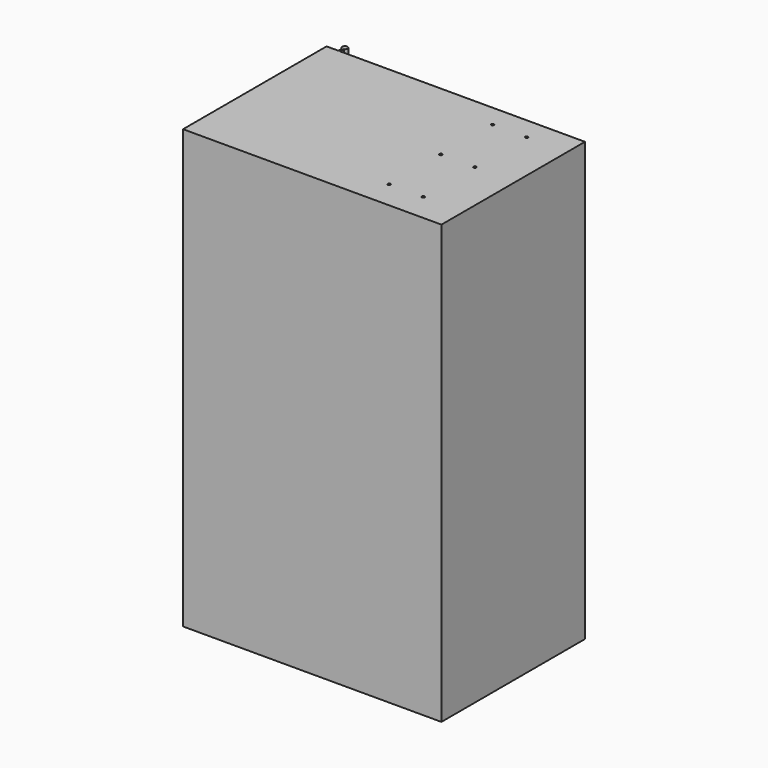
from build123d import *

# Parameters (mm, degrees)
F0_W      = 457.2
F0_H      = 774.7
F1_DEPTH  = 317.5
F2_W      = 381
F2_H      = 698.5
F3_W      = 428.625
F3_H      = 698.5
F4_DEPTH  = 298.45
F5_START  = 19.05
F5_DEPTH  = 279.4
F7_DEPTH  = 774.7
F9_D      = 4.9149
F9_DEPTH  = 38.1
F9_TIP    = 1.4765849282
F10_R     = 2.413
F11_DEPTH = 25.4


# Not quite as in the source:
# - a feature names something its author has since deleted; it is built from what else it names


with BuildPart() as f1:
    # F0 (on Front) → F1 (new body)
    with BuildSketch(Plane.XZ):
        with Locations((0, 387.35)):
            Rectangle(F0_W, F0_H)
    extrude(amount=F1_DEPTH)

    # F2 (on Front) + F3 (on Front) → F4 (cut)
    with BuildSketch(Plane.XZ):
        with Locations((0, 387.35)):
            Rectangle(F2_W, F2_H)
    with BuildSketch(Plane.XZ):
        with Locations((0, 387.35)):
            Rectangle(F3_W, F3_H)
    extrude(amount=F4_DEPTH, mode=Mode.SUBTRACT)

    # F3 (on Front) → F5 (cut)
    with BuildSketch(Plane.XZ.offset(F5_START)):
        with Locations((0, 387.35)):
            Rectangle(F3_W, F3_H)
    extrude(amount=F5_DEPTH, mode=Mode.SUBTRACT)

    # F6 (on Top) → F7 (join, through all)
    with BuildSketch(Plane.XY):
        with BuildLine():
            Line((-204.7875, 0), (-204.7875, 8.2098719395))
            ThreePointArc((-204.7875, 8.2098719395), (-206.375, 17.4625), (-207.9625, 8.2098719395))
            Line((-207.9625, 8.2098719395), (-207.9625, 0))
            Line((-207.9625, 0), (-204.7875, 0))
        make_face()
    extrude(amount=F7_DEPTH)

    # F9
    with Locations(Plane.XY.offset(774.7)):
        with Locations((96.8375, -153.9875), (157.1625, -39.6875), (157.1625, -153.9875), (96.8375, -268.2875), (96.8375, -39.6875), (157.1625, -268.2875)):
            Hole(F9_D / 2, depth=F9_DEPTH)
            with Locations((0, 0, -(F9_DEPTH + F9_TIP / 2))):  # 118° drill point
                Cone(0, F9_D / 2, F9_TIP, mode=Mode.SUBTRACT)

    # F10 (on face) → F11 (cut)
    with BuildSketch(Plane(origin=(-228.6, 0, 0), x_dir=(0, -1, 0), z_dir=(-1, 0, 0))):
        with Locations((34.925, 695.325)):
            Circle(F10_R)
        with Locations((34.925, 527.05)):
            Circle(F10_R)
        with Locations((34.925, 466.725)):
            Circle(F10_R)
        with Locations((34.925, 298.45)):
            Circle(F10_R)
        with Locations((34.925, 238.125)):
            Circle(F10_R)
        with Locations((34.925, 69.85)):
            Circle(F10_R)
        with Locations((263.525, 69.85)):
            Circle(F10_R)
        with Locations((263.525, 238.125)):
            Circle(F10_R)
        with Locations((263.525, 298.45)):
            Circle(F10_R)
        with Locations((263.525, 466.725)):
            Circle(F10_R)
        with Locations((263.525, 527.05)):
            Circle(F10_R)
        with Locations((263.525, 695.325)):
            Circle(F10_R)
    extrude(amount=-F11_DEPTH, mode=Mode.SUBTRACT)


solid = f1.part
